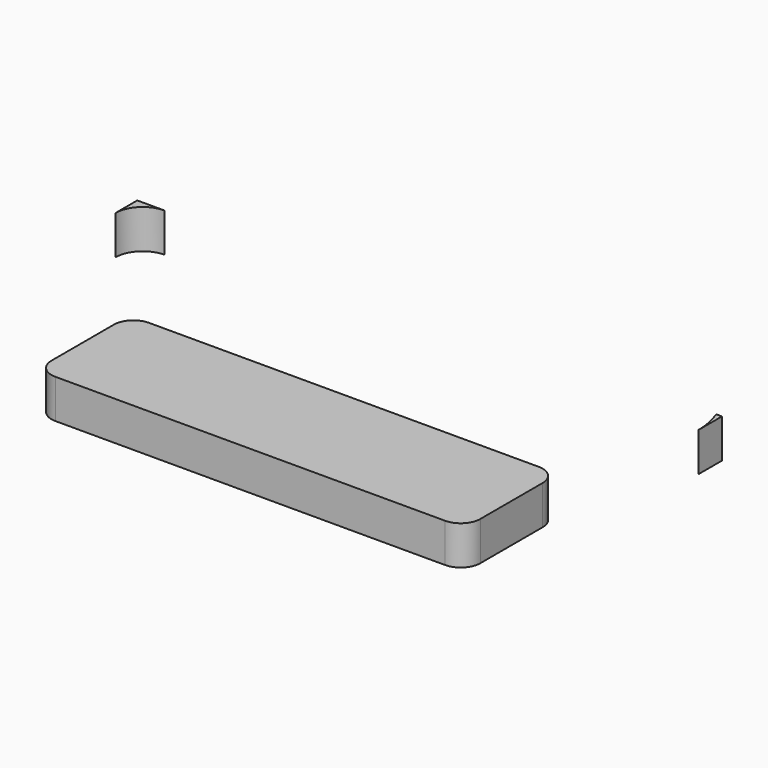
from build123d import *

# Parameters (mm, degrees)
F0_W     = 15
F0_H     = 9.9
F1_DEPTH = 1
F3_DEPTH = 25


with BuildPart() as f1:
    # F0 (on Top) → F1 (new body)
    with BuildSketch(Plane.XY):
        Rectangle(F0_W, F0_H)
    extrude(amount=F1_DEPTH)

    # F2 (on face) → F3 (cut)
    with BuildSketch(Plane.XY.offset(1)):
        with BuildLine():
            ThreePointArc((-20.5320510898, 4.95), (-18.7391055844, -1.4003756728), (-13.0962253272, -4.8208766848))
            Line((-13.0962253272, -4.8208766848), (-4.4352903374, -6.3039871505))
            ThreePointArc((-4.4352903374, -6.3039871505), (-4.2519856893, -6.1181398231), (-4, -6.05))
            Line((-4, -6.05), (6, -6.05))
            ThreePointArc((6, -6.05), (6.3495547698, -6.1924927092), (6.4998735148, -6.5387541482))
            ThreePointArc((6.4998735148, -6.5387541482), (7.1950321985, -5.8681696963), (7.4948546651, -4.95))
            Line((7.4948546651, -4.95), (3.6442812998, -4.95))
            Line((3.6442812998, -4.95), (-7.5, -4.95))
            Line((-7.5, -4.95), (-11.5771641558, -4.95))
            ThreePointArc((-11.5771641558, -4.95), (-9.480929563, -4.7024739664), (-7.5, -3.9735112293))
            Line((-7.5, -3.9735112293), (-7.5, 4.25))
            Line((-7.5, 4.25), (-7.5, 4.95))
            Line((-7.5, 4.95), (-15.3779499233, 4.95))
            Line((-15.3779499233, 4.95), (-20.5320510898, 4.95))
        make_face()
        with BuildLine():
            ThreePointArc((-4, -6.05), (-4.2519856893, -6.1181398231), (-4.4352903374, -6.3039871505))
            Line((-4.4352903374, -6.3039871505), (-1.5, -6.8066303206))
            Line((-1.5, -6.8066303206), (5.5, -6.8066303206))
            ThreePointArc((5.5, -6.8066303206), (6.0175675534, -6.738500872), (6.4998735148, -6.5387541482))
            ThreePointArc((6.4998735148, -6.5387541482), (6.3495547698, -6.1924927092), (6, -6.05))
            Line((6, -6.05), (-4, -6.05))
        make_face()
        with BuildLine():
            Line((-1.5, -6.8066303206), (-4.4352903374, -6.3039871505))
            ThreePointArc((-4.4352903374, -6.3039871505), (-4.4835520493, -6.4228095301), (-4.5, -6.55))
            Line((-4.5, -6.55), (-4.5, -8.55))
            ThreePointArc((-4.5, -8.55), (-4.3535533906, -8.9035533906), (-4, -9.05))
            Line((-4, -9.05), (-3.6551416789, -9.05))
            ThreePointArc((-3.6551416789, -9.05), (-3.1677923646, -7.4812510086), (-1.670004102, -6.8066303206))
            Line((-1.670004102, -6.8066303206), (-1.5, -6.8066303206))
        make_face()
        with BuildLine():
            ThreePointArc((-3.6128163497, 8.2415586627), (-13.2958501505, 12.8843714237), (-20.5320510898, 4.95))
            Line((-20.5320510898, 4.95), (-15.3779499233, 4.95))
            Line((-15.3779499233, 4.95), (-7.5, 4.95))
            Line((-7.5, 4.95), (-6.8, 4.95))
            Line((-6.8, 4.95), (-2.6791722048, 4.95))
            Line((-2.6791722048, 4.95), (-2.6222772219, 4.95))
            ThreePointArc((-2.6222772219, 4.95), (-2.7600582978, 5.8551715399), (-2.9890930603, 6.7416602422))
            ThreePointArc((-2.9890930603, 6.7416602422), (-3.4600899411, 7.4254340691), (-3.6128163497, 8.2415586627))
        make_face()
        with BuildLine():
            Line((5.5, -6.8066303206), (-1.5, -6.8066303206))
            Line((-1.5, -6.8066303206), (-1.3324349528, -6.8353243906))
            ThreePointArc((-1.3324349528, -6.8353243906), (-0.0653425652, -7.6128709845), (0.3151334749, -9.05))
            Line((0.3151334749, -9.05), (6, -9.05))
            ThreePointArc((6, -9.05), (6.3535533906, -8.9035533906), (6.5, -8.55))
            Line((6.5, -8.55), (6.5, -6.55))
            ThreePointArc((6.5, -6.55), (6.4999683777, -6.5443767185), (6.4998735148, -6.5387541482))
            ThreePointArc((6.4998735148, -6.5387541482), (6.0175675534, -6.738500872), (5.5, -6.8066303206))
        make_face()
        with BuildLine():
            Line((-1.3324349528, -6.8353243906), (-1.5, -6.8066303206))
            Line((-1.5, -6.8066303206), (-1.670004102, -6.8066303206))
            ThreePointArc((-1.670004102, -6.8066303206), (-3.1677923646, -7.4812510086), (-3.6551416789, -9.05))
            Line((-3.6551416789, -9.05), (0.3151334749, -9.05))
            ThreePointArc((0.3151334749, -9.05), (-0.0653425652, -7.6128709845), (-1.3324349528, -6.8353243906))
        make_face()
        with BuildLine():
            ThreePointArc((-2.9890930603, 6.7416602422), (-3.2670458238, 7.5057102466), (-3.6128163497, 8.2415586627))
            ThreePointArc((-3.6128163497, 8.2415586627), (-3.4600899411, 7.4254340691), (-2.9890930603, 6.7416602422))
        make_face()
        with BuildLine():
            ThreePointArc((-1.387329764, 6.206187349), (-0.2636271595, 9.6692156863), (-3.6128163497, 8.2415586627))
            ThreePointArc((-3.6128163497, 8.2415586627), (-3.2670458238, 7.5057102466), (-2.9890930603, 6.7416602422))
            ThreePointArc((-2.9890930603, 6.7416602422), (-2.3538634279, 6.3354920093), (-1.6133969785, 6.1933696794))
            Line((-1.6133969785, 6.1933696794), (5.5, 6.1933696794))
            ThreePointArc((5.5, 6.1933696794), (6.6150648768, 5.853679988), (7.3513537096, 4.95))
            Line((7.3513537096, 4.95), (7.5, 4.95))
            Line((7.5, 4.95), (146.3048853708, 4.95))
            ThreePointArc((146.3048853708, 4.95), (137.3193168194, 13.4405318382), (145.2875829058, 22.8923204871))
            Line((145.2875829058, 22.8923204871), (-1.387329764, 6.206187349))
        make_face()
        with BuildLine():
            ThreePointArc((-1.6133969785, 6.1933696794), (-2.3538634279, 6.3354920093), (-2.9890930603, 6.7416602422))
            ThreePointArc((-2.9890930603, 6.7416602422), (-2.7600582978, 5.8551715399), (-2.6222772219, 4.95))
            Line((-2.6222772219, 4.95), (7.3513537096, 4.95))
            ThreePointArc((7.3513537096, 4.95), (6.6150648768, 5.853679988), (5.5, 6.1933696794))
            Line((5.5, 6.1933696794), (-1.6133969785, 6.1933696794))
        make_face()
        with BuildLine():
            ThreePointArc((-3.6551416789, -9.05), (-1.670004102, -10.8066303206), (0.3151334749, -9.05))
            Line((0.3151334749, -9.05), (-3.6551416789, -9.05))
        make_face()
        with BuildLine():
            Line((-2.6791722048, 4.95), (-6.8, 4.95))
            ThreePointArc((-6.8, 4.95), (-7.2949747468, 4.7449747468), (-7.5, 4.25))
            Line((-7.5, 4.25), (-7.5, -3.9735112293))
            ThreePointArc((-7.5, -3.9735112293), (-5.8655999589, -2.9054320085), (-4.5, -1.5100132654))
            Line((-4.5, -1.5100132654), (-4.5, 0.45))
            ThreePointArc((-4.5, 0.45), (-4.3535533906, 0.8035533906), (-4, 0.95))
            Line((-4, 0.95), (-3.1279038332, 0.95))
            ThreePointArc((-3.1279038332, 0.95), (-2.6482176652, 2.9213217609), (-2.6222772219, 4.95))
            Line((-2.6222772219, 4.95), (-2.6791722048, 4.95))
        make_face()
        with BuildLine():
            Line((7.3513537096, 4.95), (-2.6222772219, 4.95))
            ThreePointArc((-2.6222772219, 4.95), (-2.6482176652, 2.9213217609), (-3.1279038332, 0.95))
            Line((-3.1279038332, 0.95), (6, 0.95))
            ThreePointArc((6, 0.95), (6.3535533906, 0.8035533906), (6.5, 0.45))
            Line((6.5, 0.45), (6.5, -1.55))
            ThreePointArc((6.5, -1.55), (6.3535533906, -1.9035533906), (6, -2.05))
            Line((6, -2.05), (-4, -2.05))
            ThreePointArc((-4, -2.05), (-4.3535533906, -1.9035533906), (-4.5, -1.55))
            Line((-4.5, -1.55), (-4.5, -1.5100132654))
            ThreePointArc((-4.5, -1.5100132654), (-5.8655999589, -2.9054320085), (-7.5, -3.9735112293))
            Line((-7.5, -3.9735112293), (-7.5, -4.95))
            Line((-7.5, -4.95), (3.6442812998, -4.95))
            Line((3.6442812998, -4.95), (7.4948546651, -4.95))
            ThreePointArc((7.4948546651, -4.95), (7.4987132524, -4.8783613101), (7.5, -4.8066303206))
            Line((7.5, -4.8066303206), (7.5, 4.1933696794))
            ThreePointArc((7.5, 4.1933696794), (7.4624866139, 4.5789164216), (7.3513537096, 4.95))
        make_face()
        with BuildLine():
            ThreePointArc((7.5, -4.8066303206), (7.4987132524, -4.8783613101), (7.4948546651, -4.95))
            Line((7.4948546651, -4.95), (7.5, -4.95))
            Line((7.5, -4.95), (7.5, -4.8066303206))
        make_face()
        with BuildLine():
            Line((-7.5, -4.95), (-7.5, -3.9735112293))
            ThreePointArc((-7.5, -3.9735112293), (-9.480929563, -4.7024739664), (-11.5771641558, -4.95))
            Line((-11.5771641558, -4.95), (-7.5, -4.95))
        make_face()
        with BuildLine():
            ThreePointArc((-4, -13.05), (-4.3535533906, -13.1964466094), (-4.5, -13.55))
            Line((-4.5, -13.55), (-4.5, -15.55))
            ThreePointArc((-4.5, -15.55), (-4.3535533906, -15.9035533906), (-4, -16.05))
            Line((-4, -16.05), (6, -16.05))
            ThreePointArc((6, -16.05), (6.3535533906, -15.9035533906), (6.5, -15.55))
            Line((6.5, -15.55), (6.5, -13.55))
            ThreePointArc((6.5, -13.55), (6.3535533906, -13.1964466094), (6, -13.05))
            Line((6, -13.05), (-4, -13.05))
        make_face()
    extrude(amount=-F3_DEPTH, mode=Mode.SUBTRACT)


solid = f1.part
